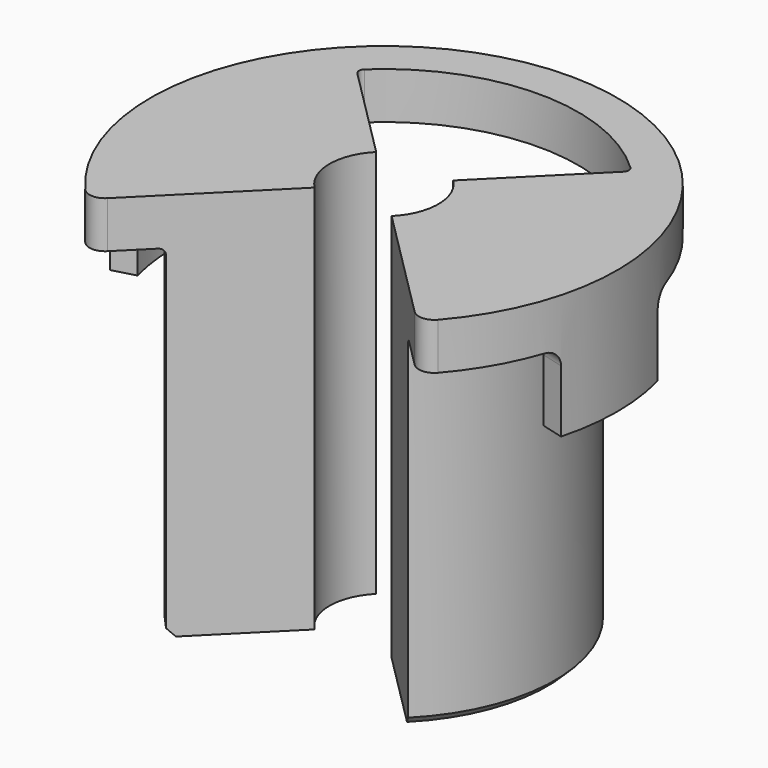
from build123d import *

# Parameters (mm, degrees)
F0_R      = 11
F0_R_2    = 3.5
F1_DEPTH  = 25
F2_R      = 15
F2_R_2    = 3.5
F3_DEPTH  = 8
F4_R      = 13.5
F4_R_2    = 11
F5_DEPTH  = 5
F6_R      = 0.4
F8_DEPTH  = 25
F10_DEPTH = 5
F12_R     = 1
F13_SIZE  = 0.5
F15_DEPTH = 3
F16_R     = 0.4


# Not quite as in the source:
# - a feature of the source that left no trace in its solid (it failed there, or was rolled back) is left out


with BuildPart() as f1:
    # F0 (on Top) → F1 (new body)
    with BuildSketch(Plane.XY):
        Circle(F0_R)
        Circle(F0_R_2, mode=Mode.SUBTRACT)
    extrude(amount=-F1_DEPTH)

    # F2 (on Top) → F3 (join)
    with BuildSketch(Plane.XY):
        Circle(F2_R)
        Circle(F2_R_2, mode=Mode.SUBTRACT)
    extrude(amount=-F3_DEPTH)

    # F4 (on face) → F5 (cut)
    with BuildSketch(Plane(origin=(0, 0, -8), x_dir=(1, 0, 0), z_dir=(0, 0, -1))):
        Circle(F4_R)
        Circle(F4_R_2, mode=Mode.SUBTRACT)
    extrude(amount=-F5_DEPTH, mode=Mode.SUBTRACT)

    # F6
    f6_edges = [f1.edges().sort_by_distance(p)[0] for p in [
        (-13.5, 0, -3),
    ]]
    fillet(f6_edges, radius=F6_R)

    # F7 (on Top) → F8 (cut)
    with BuildSketch(Plane.XY):
        with BuildLine():
            ThreePointArc((-2.4748737342, 2.4748737342), (0, 3.5), (2.4748737342, 2.4748737342))
            Line((2.4748737342, 2.4748737342), (10.6066017178, 10.6066017178))
            ThreePointArc((10.6066017178, 10.6066017178), (0, 15), (-10.6066017178, 10.6066017178))
            Line((-10.6066017178, 10.6066017178), (-2.4748737342, 2.4748737342))
        make_face()
        with BuildLine():
            Line((10.6066017178, -10.6066017178), (2.4748737342, -2.4748737342))
            ThreePointArc((2.4748737342, -2.4748737342), (0, -3.5), (-2.4748737342, -2.4748737342))
            Line((-2.4748737342, -2.4748737342), (-10.6066017178, -10.6066017178))
            ThreePointArc((-10.6066017178, -10.6066017178), (0, -15), (10.6066017178, -10.6066017178))
        make_face()
    extrude(amount=-F8_DEPTH, mode=Mode.SUBTRACT)

    # F9 (on face) → F10 (cut, through all)
    with BuildSketch(Plane(origin=(0, 0, -8), x_dir=(1, 0, 0), z_dir=(0, 0, -1))):
        with BuildLine():
            ThreePointArc((-10.6251840892, 2.8470094961), (0, 11), (10.6251840892, 2.8470094961))
            Line((10.6251840892, 2.8470094961), (15.4548132206, 4.1411047216))
            ThreePointArc((15.4548132206, 4.1411047216), (0, 16), (-15.4548132206, 4.1411047216))
            Line((-15.4548132206, 4.1411047216), (-10.6251840892, 2.8470094961))
        make_face()
        with BuildLine():
            Line((15.4548132206, -4.1411047216), (10.6251840892, -2.8470094961))
            ThreePointArc((10.6251840892, -2.8470094961), (0, -11), (-10.6251840892, -2.8470094961))
            Line((-10.6251840892, -2.8470094961), (-15.4548132206, -4.1411047216))
            ThreePointArc((-15.4548132206, -4.1411047216), (0, -16), (15.4548132206, -4.1411047216))
        make_face()
    extrude(amount=-F10_DEPTH, mode=Mode.SUBTRACT)

    # F12 (call 1 of 6: OpenCascade refuses the feature's edges together)
    f12_edges = [f1.edges().sort_by_distance(p)[0] for p in [
        (10.606602, -10.606602, -1.5),
    ]]
    fillet(f12_edges, radius=F12_R)

    # F12#2 (call 2 of 6)
    f12_2_edges = [f1.edges().sort_by_distance(p)[0] for p in [
        (-10.606602, -10.606602, -1.5),
    ]]
    fillet(f12_2_edges, radius=F12_R)

    # F12#3 (call 3 of 6)
    f12_3_edges = [f1.edges().sort_by_distance(p)[0] for p in [
        (13.571258, -3.636408, -3),
    ]]
    fillet(f12_3_edges, radius=F12_R)

    # F12#4 (call 4 of 6)
    f12_4_edges = [f1.edges().sort_by_distance(p)[0] for p in [
        (13.571258, 3.636408, -3),
    ]]
    fillet(f12_4_edges, radius=F12_R)

    # F12#5 (call 5 of 6)
    f12_5_edges = [f1.edges().sort_by_distance(p)[0] for p in [
        (-13.571258, -3.636408, -3),
    ]]
    fillet(f12_5_edges, radius=F12_R)

    # F12#6 (call 6 of 6)
    f12_6_edges = [f1.edges().sort_by_distance(p)[0] for p in [
        (-13.571258, 3.636408, -3),
    ]]
    fillet(f12_6_edges, radius=F12_R)

    # F13
    f13_edges = [f1.edges().sort_by_distance(p)[0] for p in [
        (-11, 0, -25),
        (11, 0, -25),
    ]]
    chamfer(f13_edges, length=F13_SIZE)

    # F14 (on Top) → F15 (join)
    with BuildSketch(Plane.XY):
        with BuildLine():
            Line((12.5, 0), (15, 0))
            ThreePointArc((15, 0), (0, 15), (-15, 0))
            Line((-15, 0), (-12.5, 0))
            ThreePointArc((-12.5, 0), (0, 12.5), (12.5, 0))
        make_face()
    extrude(amount=-F15_DEPTH)

    # F16
    f16_edges = [f1.edges().sort_by_distance(p)[0] for p in [
        (11, 0, -3),
        (-11, 0, -3),
        (-8.838835, 8.838835, -1.5),
        (8.838835, 8.838835, -1.5),
    ]]
    fillet(f16_edges, radius=F16_R)


solid = f1.part
